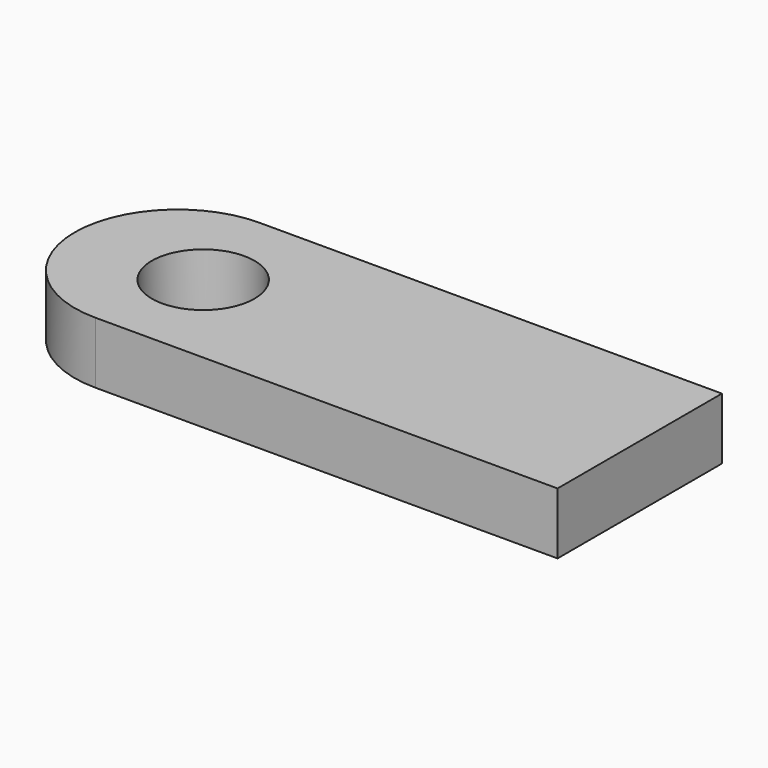
from build123d import *

# Parameters (mm, degrees)
F0_W     = 13.97
F0_H     = 5.08
F1_DEPTH = 1.524
F2_R     = 1.27
F3_DEPTH = 25.4
F4_R     = 2.53999


# Not quite as in the source:
# - a fillet or chamfer is up to 0.001 mm smaller than in the source, because OpenCascade refuses the exact size


with BuildPart() as f1:
    # F0 (on Top) → F1 (new body)
    with BuildSketch(Plane.XY):
        with Locations((6.985, 2.54)):
            Rectangle(F0_W, F0_H)
    extrude(amount=F1_DEPTH)

    # F2 (on face) → F3 (cut)
    with BuildSketch(Plane.XY.offset(1.524)):
        with Locations((3.175, 2.54)):
            Circle(F2_R)
    extrude(amount=-F3_DEPTH, mode=Mode.SUBTRACT)

    # F4 (radius 2.54 in the source; OpenCascade refuses exactly that, so slightly less here)
    f4_edges = [f1.edges().sort_by_distance(p)[0] for p in [
        (0, 0, 0.762),
        (0, 5.08, 0.762),
    ]]
    fillet(f4_edges, radius=F4_R)


solid = f1.part
